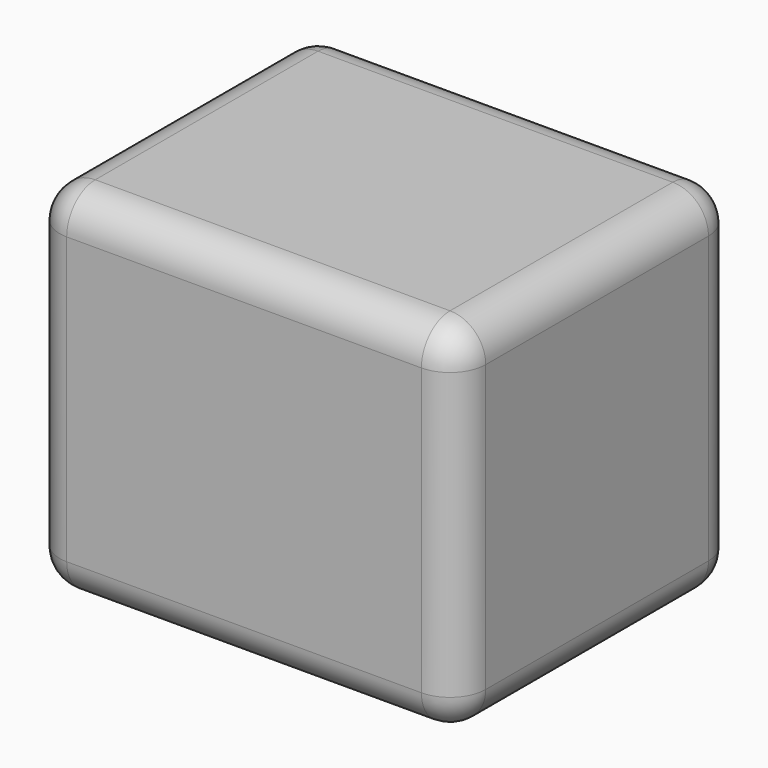
from build123d import *

# Parameters (mm, degrees)
F0_W         = 60.5695545673
F0_H         = 49.7252251953
F1_DEPTH     = 50.8
F2_R         = 5.08
F3_R         = 5.08
F4_T1_DEPTH  = 40.64
F4_S5_W      = 5.08
F4_S5_H      = 5.08
F4_T6_DEPTH  = 5.08
F4_S11_W     = 5.08
F4_S11_H     = 5.08
F4_T12_DEPTH = 5.08
F4_S17_W     = 5.08
F4_S17_H     = 5.08
F4_T18_DEPTH = 5.08
F4_S23_W     = 5.08
F4_S23_H     = 5.08
F4_T24_DEPTH = 5.08
F4_S29_W     = 5.08
F4_S29_H     = 5.08
F4_T30_DEPTH = 5.08
F4_S35_W     = 5.08
F4_S35_H     = 5.08
F4_T36_DEPTH = 5.08
F4_S41_W     = 5.08
F4_S41_H     = 5.08
F4_T42_DEPTH = 5.08
F4_S47_W     = 5.08
F4_S47_H     = 5.08
F4_T48_DEPTH = 5.08


# Not quite as in the source:
# - a fillet or chamfer that OpenCascade refuses, or shapes differently, is made with other operations: its cross-section is extruded or revolved along the edge and cut away or added


with BuildPart() as f1:
    # F0 (on Top) → F1 (new body)
    with BuildSketch(Plane.XY):
        with Locations((3.8351900876, -0.2644965425)):
            Rectangle(F0_W, F0_H)
    extrude(amount=F1_DEPTH)

    # F2
    f2_edges = [f1.edges().sort_by_distance(p)[0] for p in [
        (3.83519, -25.127109, 50.8),
        (-26.449587, -0.264497, 50.8),
        (3.83519, 24.598116, 50.8),
        (34.119967, -0.264497, 50.8),
    ]]
    fillet(f2_edges, radius=F2_R)

    # F3
    f3_edges = [f1.edges().sort_by_distance(p)[0] for p in [
        (3.83519, -25.127109, 0),
        (34.119967, -0.264497, 0),
        (3.83519, 24.598116, 0),
        (-26.449587, -0.264497, 0),
    ]]
    fillet(f3_edges, radius=F3_R)

    # F4: fillet of radius 5.08 on 4 edges, made by hand

    # F4_s2 → F4_t1 (cut)
    with BuildSketch(Plane.XY.offset(5.08)):
        with BuildLine():
            ThreePointArc((-21.3695871961, 24.5981160551), (-24.9616896445, 23.1102185036), (-26.4495871961, 19.5181160551))
            Line((-26.4495871961, 19.5181160551), (-26.4495871961, 24.5981160551))
            Line((-26.4495871961, 24.5981160551), (-21.3695871961, 24.5981160551))
        make_face()
        with BuildLine():
            ThreePointArc((-26.4495871961, -20.0471091402), (-24.9616896445, -23.6392115886), (-21.3695871961, -25.1271091402))
            Line((-21.3695871961, -25.1271091402), (-26.4495871961, -25.1271091402))
            Line((-26.4495871961, -25.1271091402), (-26.4495871961, -20.0471091402))
        make_face()
        with BuildLine():
            ThreePointArc((29.0399673712, 24.5981160551), (32.6320698197, 23.1102185036), (34.1199673712, 19.5181160551))
            Line((34.1199673712, 19.5181160551), (34.1199673712, 24.5981160551))
            Line((34.1199673712, 24.5981160551), (29.0399673712, 24.5981160551))
        make_face()
        with BuildLine():
            ThreePointArc((34.1199673712, -20.0471091402), (32.6320698197, -23.6392115886), (29.0399673712, -25.1271091402))
            Line((29.0399673712, -25.1271091402), (34.1199673712, -25.1271091402))
            Line((34.1199673712, -25.1271091402), (34.1199673712, -20.0471091402))
        make_face()
    extrude(amount=F4_T1_DEPTH, mode=Mode.SUBTRACT)


with BuildPart() as f4_tool4:
    # F4_s5 → F4_t6 (new body)
    with BuildSketch(Plane.YZ.offset(29.0399673712)):
        with Locations((-22.5871091402, 2.54)):
            Rectangle(F4_S5_W, F4_S5_H)
    extrude(amount=F4_T6_DEPTH)

    # F4_s7 → F4_t8 (revolve, cut)
    with BuildSketch(Plane(origin=(29.0399673712, -20.0471091402, 5.08), x_dir=(0, 0.7071067812, 0.7071067812), z_dir=(0, 0.7071067812, -0.7071067812))):
        with BuildLine():
            ThreePointArc((0, -5.08), (5.08, 0), (0, 5.08))
            Line((0, 5.08), (0, -5.08))
        make_face()
    revolve(axis=Axis((29.0399673712, -20.0471091402, 5.08), (1, 0, 0)), mode=Mode.SUBTRACT)


with BuildPart() as f1_1:
    add(f1.part)

    # F4_t3: cut F4_tool4
    add(f4_tool4.part, mode=Mode.SUBTRACT)


with BuildPart() as f4_tool10:
    # F4_s11 → F4_t12 (new body)
    with BuildSketch(Plane.YZ.offset(29.0399673712)):
        with Locations((-22.5871091402, 48.26)):
            Rectangle(F4_S11_W, F4_S11_H)
    extrude(amount=F4_T12_DEPTH)

    # F4_s13 → F4_t14 (revolve, cut)
    with BuildSketch(Plane(origin=(29.0399673712, -20.0471091402, 45.72), x_dir=(0, 0.7071067812, -0.7071067812), z_dir=(0, -0.7071067812, -0.7071067812))):
        with BuildLine():
            ThreePointArc((0, -5.08), (5.08, 0), (0, 5.08))
            Line((0, 5.08), (0, -5.08))
        make_face()
    revolve(axis=Axis((29.0399673712, -20.0471091402, 45.72), (1, 0, 0)), mode=Mode.SUBTRACT)


with BuildPart() as f1_2:
    add(f1_1.part)

    # F4_t9: cut F4_tool10
    add(f4_tool10.part, mode=Mode.SUBTRACT)


with BuildPart() as f4_tool16:
    # F4_s17 → F4_t18 (new body)
    with BuildSketch(Plane.XZ.offset(-19.5181160551)):
        with Locations((31.5799673712, 2.54)):
            Rectangle(F4_S17_W, F4_S17_H)
    extrude(amount=-F4_T18_DEPTH)

    # F4_s19 → F4_t20 (revolve, cut)
    with BuildSketch(Plane(origin=(29.0399673712, 19.5181160551, 5.08), x_dir=(-0.7071067812, 0, 0.7071067812), z_dir=(-0.7071067812, 0, -0.7071067812))):
        with BuildLine():
            ThreePointArc((0, -5.08), (5.08, 0), (0, 5.08))
            Line((0, 5.08), (0, -5.08))
        make_face()
    revolve(axis=Axis((29.0399673712, 19.5181160551, 5.08), (0, 1, 0)), mode=Mode.SUBTRACT)


with BuildPart() as f1_3:
    add(f1_2.part)

    # F4_t15: cut F4_tool16
    add(f4_tool16.part, mode=Mode.SUBTRACT)


with BuildPart() as f4_tool22:
    # F4_s23 → F4_t24 (new body)
    with BuildSketch(Plane.XZ.offset(-19.5181160551)):
        with Locations((31.5799673712, 48.26)):
            Rectangle(F4_S23_W, F4_S23_H)
    extrude(amount=-F4_T24_DEPTH)

    # F4_s25 → F4_t26 (revolve, cut)
    with BuildSketch(Plane(origin=(29.0399673712, 19.5181160551, 45.72), x_dir=(-0.7071067812, 0, -0.7071067812), z_dir=(0.7071067812, 0, -0.7071067812))):
        with BuildLine():
            ThreePointArc((0, -5.08), (5.08, 0), (0, 5.08))
            Line((0, 5.08), (0, -5.08))
        make_face()
    revolve(axis=Axis((29.0399673712, 19.5181160551, 45.72), (0, 1, 0)), mode=Mode.SUBTRACT)


with BuildPart() as f1_4:
    add(f1_3.part)

    # F4_t21: cut F4_tool22
    add(f4_tool22.part, mode=Mode.SUBTRACT)


with BuildPart() as f4_tool28:
    # F4_s29 → F4_t30 (new body)
    with BuildSketch(Plane.YZ.offset(-21.3695871961)):
        with Locations((-22.5871091402, 2.54)):
            Rectangle(F4_S29_W, F4_S29_H)
    extrude(amount=-F4_T30_DEPTH)

    # F4_s31 → F4_t32 (revolve, cut)
    with BuildSketch(Plane(origin=(-21.3695871961, -20.0471091402, 5.08), x_dir=(0, 0.7071067812, 0.7071067812), z_dir=(0, -0.7071067812, 0.7071067812))):
        with BuildLine():
            ThreePointArc((0, -5.08), (5.08, 0), (0, 5.08))
            Line((0, 5.08), (0, -5.08))
        make_face()
    revolve(axis=Axis((-21.3695871961, -20.0471091402, 5.08), (-1, 0, 0)), mode=Mode.SUBTRACT)


with BuildPart() as f1_5:
    add(f1_4.part)

    # F4_t27: cut F4_tool28
    add(f4_tool28.part, mode=Mode.SUBTRACT)


with BuildPart() as f4_tool34:
    # F4_s35 → F4_t36 (new body)
    with BuildSketch(Plane.YZ.offset(-21.3695871961)):
        with Locations((-22.5871091402, 48.26)):
            Rectangle(F4_S35_W, F4_S35_H)
    extrude(amount=-F4_T36_DEPTH)

    # F4_s37 → F4_t38 (revolve, cut)
    with BuildSketch(Plane(origin=(-21.3695871961, -20.0471091402, 45.72), x_dir=(0, 0.7071067812, -0.7071067812), z_dir=(0, 0.7071067812, 0.7071067812))):
        with BuildLine():
            ThreePointArc((0, -5.08), (5.08, 0), (0, 5.08))
            Line((0, 5.08), (0, -5.08))
        make_face()
    revolve(axis=Axis((-21.3695871961, -20.0471091402, 45.72), (-1, 0, 0)), mode=Mode.SUBTRACT)


with BuildPart() as f1_6:
    add(f1_5.part)

    # F4_t33: cut F4_tool34
    add(f4_tool34.part, mode=Mode.SUBTRACT)


with BuildPart() as f4_tool40:
    # F4_s41 → F4_t42 (new body)
    with BuildSketch(Plane.XZ.offset(-19.5181160551)):
        with Locations((-23.9095871961, 2.54)):
            Rectangle(F4_S41_W, F4_S41_H)
    extrude(amount=-F4_T42_DEPTH)

    # F4_s43 → F4_t44 (revolve, cut)
    with BuildSketch(Plane(origin=(-21.3695871961, 19.5181160551, 5.08), x_dir=(0.7071067812, 0, 0.7071067812), z_dir=(-0.7071067812, 0, 0.7071067812))):
        with BuildLine():
            ThreePointArc((0, -5.08), (5.08, 0), (0, 5.08))
            Line((0, 5.08), (0, -5.08))
        make_face()
    revolve(axis=Axis((-21.3695871961, 19.5181160551, 5.08), (0, 1, 0)), mode=Mode.SUBTRACT)


with BuildPart() as f1_7:
    add(f1_6.part)

    # F4_t39: cut F4_tool40
    add(f4_tool40.part, mode=Mode.SUBTRACT)


with BuildPart() as f4_tool46:
    # F4_s47 → F4_t48 (new body)
    with BuildSketch(Plane.XZ.offset(-19.5181160551)):
        with Locations((-23.9095871961, 48.26)):
            Rectangle(F4_S47_W, F4_S47_H)
    extrude(amount=-F4_T48_DEPTH)

    # F4_s49 → F4_t50 (revolve, cut)
    with BuildSketch(Plane(origin=(-21.3695871961, 19.5181160551, 45.72), x_dir=(0.7071067812, 0, -0.7071067812), z_dir=(0.7071067812, 0, 0.7071067812))):
        with BuildLine():
            ThreePointArc((0, -5.08), (5.08, 0), (0, 5.08))
            Line((0, 5.08), (0, -5.08))
        make_face()
    revolve(axis=Axis((-21.3695871961, 19.5181160551, 45.72), (0, 1, 0)), mode=Mode.SUBTRACT)


with BuildPart() as f1_8:
    add(f1_7.part)

    # F4_t45: cut F4_tool46
    add(f4_tool46.part, mode=Mode.SUBTRACT)


solid = f1_8.part
